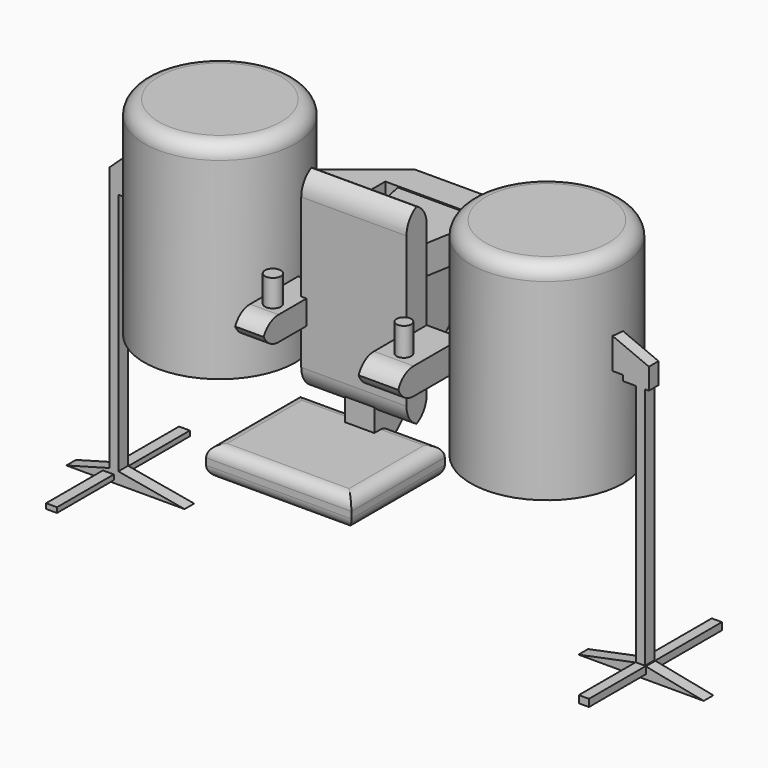
from build123d import *

# Parameters (mm, degrees)
F0_R         = 160.6336286285
F1_DEPTH     = 218.44
F0_R_2       = 159.7328245583
F3_DEPTH     = 63.5
F4_W         = 221.9782620668
F4_H         = 414.4903868437
F5_DEPTH     = 53.34
F6_T1_DEPTH  = 467.2623600039
F8_DEPTH     = 60.96
F4_W_2       = 306.4478710294
F4_H_2       = 62.861084938
F9_DEPTH     = 246.38
F10_R        = 24.5284097937
F11_W        = 61.5484267473
F11_H        = 264.6007202566
F12_DEPTH    = 287.782
F13_SIZE     = 205.74
F14_SIZE     = 81.28
F19_W        = 18.9964473248
F19_H        = 513.7299746275
F20_DEPTH    = 25.4
F21_W        = 22.9676365852
F21_H        = 10.7182264328
F22_DEPTH    = 175.26
F21_W_2      = 21.4364528656
F21_H_2      = 15.3118371964
F23_W        = 83.6651213467
F23_H        = 56.2124997377
F23_W_2      = 60.1342916489
F23_H_2      = 50.9834252298
F24_DEPTH    = 170.18
F25_T1_DEPTH = 274.7578773438
F25_T3_DEPTH = 298.2887070417
F26_R        = 30.6605122421
F26_2_R      = 30.6605122421
F27_R        = 16.7759014108
F28_DEPTH    = 93.722416088
F27_R_2      = 15.45819276


# Not quite as in the source:
# - a fillet or chamfer that OpenCascade refuses, or shapes differently, is made with other operations: its cross-section is extruded or revolved along the edge and cut away or added
# - the program builds the solid bodies; features that only make, move or delete a surface that nothing else refers to are left out


with BuildPart() as f1:
    # F0 (on Top) → F1 (new body, symmetric)
    with BuildSketch(Plane.XY):
        with Locations((167.6235944033, 0)):
            Circle(F0_R)
    extrude(amount=F1_DEPTH, both=True)

    # F26
    f26_edges = [f1.edges().sort_by_distance(p)[0] for p in [
        (6.989966, 0, 218.44),
    ]]
    fillet(f26_edges, radius=F26_R)


with BuildPart() as f1b:
    # F0 (on Top) → F1, piece 2 (new body, symmetric)
    with BuildSketch(Plane.XY):
        with Locations((-522.2776532173, 0)):
            Circle(F0_R_2)
    extrude(amount=F1_DEPTH, both=True)

    # F26#2
    f26_2_edges = [f1b.edges().sort_by_distance(p)[0] for p in [
        (-682.010478, 0, 218.44),
    ]]
    fillet(f26_2_edges, radius=F26_2_R)


with BuildPart() as f3:
    # F2 (on Top) → F3 (new body)
    with BuildSketch(Plane.XY):
        Polygon((-300.143301487, 237.2024357319), (-437.6519620419, 127.195507288), (-432.7409267426, 106.5692082047), (-312.0444483441, 106.5692082047), (-312.0444483441, 173.3591258526), (-42.8056791425, 173.3591258526), (-42.8056791425, 96.7471674085), (99.6140241623, 96.7471674085), (99.6140241623, 131.1243325472), (-56.5565414727, 237.2024357319), align=None)
    extrude(amount=F3_DEPTH)


with BuildPart() as f5:
    # F4 (on Front) → F5 (new body)
    with BuildSketch(Plane.XZ):
        with Locations((-197.0118135214, -29.95724231)):
            Rectangle(F4_W, F4_H)
    extrude(amount=F5_DEPTH)

    # F6: fillet of radius 49.0568195874 on 4 edges, made by hand

    # F6_s2 → F6_t1 (cut)
    with BuildSketch(Plane.YZ.offset(-430.6429935234)):
        with BuildLine():
            ThreePointArc((-49.0568195874, -237.2024357319), (-14.3684097937, -222.8340259382), (0, -188.1456161445))
            Line((0, -188.1456161445), (0, -237.2024357319))
            Line((0, -237.2024357319), (-49.0568195874, -237.2024357319))
        make_face()
        with BuildLine():
            ThreePointArc((-4.2831804126, -237.2024357319), (-38.9715902063, -222.8340259382), (-53.34, -188.1456161445))
            Line((-53.34, -188.1456161445), (-53.34, -237.2024357319))
            Line((-53.34, -237.2024357319), (-4.2831804126, -237.2024357319))
        make_face()
        with BuildLine():
            ThreePointArc((-4.2831804126, 177.2879511118), (-38.9715902063, 162.9195413181), (-53.34, 128.2311315244))
            Line((-53.34, 128.2311315244), (-53.34, 177.2879511118))
            Line((-53.34, 177.2879511118), (-4.2831804126, 177.2879511118))
        make_face()
        with BuildLine():
            ThreePointArc((-49.0568195874, 177.2879511118), (-14.3684097937, 162.9195413181), (0, 128.2311315244))
            Line((0, 128.2311315244), (0, 177.2879511118))
            Line((0, 177.2879511118), (-49.0568195874, 177.2879511118))
        make_face()
    extrude(amount=F6_T1_DEPTH, mode=Mode.SUBTRACT)

    # F23 (on Front) → F24 (join)
    with BuildSketch(Plane.XZ):
        with Locations((-53.6179151386, -87.4198973179)):
            Rectangle(F23_W, F23_H)
        with Locations((-326.8368244171, -82.1908283979)):
            Rectangle(F23_W_2, F23_H_2)
    extrude(amount=F24_DEPTH)

    # F25: fillet of radius 42.924717139 on 4 edges, made by hand

    # F25_s2 → F25_t1 (cut)
    with BuildSketch(Plane.YZ.offset(-464.215763089)):
        with BuildLine():
            ThreePointArc((-127.255282861, -56.699115783), (-157.6076414305, -69.2714743525), (-170.18, -99.623832922))
            Line((-170.18, -99.623832922), (-170.18, -56.699115783))
            Line((-170.18, -56.699115783), (-127.255282861, -56.699115783))
        make_face()
        with BuildLine():
            ThreePointArc((-127.255282861, -107.6825410128), (-157.6076414305, -95.1101824433), (-170.18, -64.7578238738))
            Line((-170.18, -64.7578238738), (-170.18, -107.6825410128))
            Line((-170.18, -107.6825410128), (-127.255282861, -107.6825410128))
        make_face()
    extrude(amount=F25_T1_DEPTH, mode=Mode.SUBTRACT)

    # F25_s4 → F25_t3 (cut)
    with BuildSketch(Plane.YZ.offset(-202.7622686594)):
        with BuildLine():
            ThreePointArc((-170.18, -102.238364588), (-157.6076414305, -71.8860060185), (-127.255282861, -59.313647449))
            Line((-127.255282861, -59.313647449), (-170.18, -59.313647449))
            Line((-170.18, -59.313647449), (-170.18, -102.238364588))
        make_face()
        with BuildLine():
            ThreePointArc((-127.255282861, -115.5261471868), (-157.6076414305, -102.9537886173), (-170.18, -72.6014300478))
            Line((-170.18, -72.6014300478), (-170.18, -115.5261471868))
            Line((-170.18, -115.5261471868), (-127.255282861, -115.5261471868))
        make_face()
    extrude(amount=F25_T3_DEPTH, mode=Mode.SUBTRACT)


with BuildPart() as f8:
    # F7 (on Top) → F8 (new body)
    with BuildSketch(Plane.XY):
        Polygon((-98.7913385034, 196.9104707241), (-290.3212606907, 192.9816454649), (-244.1576421261, -9.3525238335), (-134.1507136822, -9.3525238335), align=None)
    extrude(amount=F8_DEPTH)


with BuildPart() as f9:
    # F4 (on Front) → F9 (new body)
    with BuildSketch(Plane.XZ):
        with Locations((-201.0610103607, -299.5766699314)):
            Rectangle(F4_W_2, F4_H_2)
    extrude(amount=F9_DEPTH)

    # F10
    f10_edges = [f9.edges().sort_by_distance(p)[0] for p in [
        (-354.284946, -123.19, -268.146127),
        (-354.284946, -123.19, -331.007212),
        (-47.837075, -123.19, -268.146127),
        (-47.837075, -123.19, -331.007212),
        (-201.06101, -246.38, -268.146127),
        (-201.06101, -246.38, -331.007212),
        (-201.06101, 0, -268.146127),
        (-201.06101, 0, -331.007212),
    ]]
    fillet(f10_edges, radius=F10_R)


with BuildPart() as f12:
    # F11 (on Top) → F12 (new body)
    with BuildSketch(Plane.XY):
        with Locations((-194.3048760295, 91.1482293159)):
            Rectangle(F11_W, F11_H)
    extrude(amount=-F12_DEPTH)

    # F13
    f13_edges = [f12.edges().sort_by_distance(p)[0] for p in [
        (-194.304876, 223.448589, -287.782),
    ]]
    chamfer(f13_edges, length=F13_SIZE)

    # F14
    f14_edges = [f12.edges().sort_by_distance(p)[0] for p in [
        (-194.304876, 223.448589, -82.042),
    ]]
    chamfer(f14_edges, length=F14_SIZE)


with BuildPart() as f20:
    # F19 (on Front) → F20 (new body)
    with BuildSketch(Plane.XZ):
        Polygon((-662.3982787132, 0), (-672.3094582558, 90.7716751099), (-735.0803017616, 32.9563878477), (-735.0803017616, -11.643961072), (-716.0838544369, -11.643961072), (-697.0874071121, -11.643961072), (-697.0874071121, 0), align=None)
        with Locations((-725.5820780993, -268.5089483857)):
            Rectangle(F19_W, F19_H)
        Polygon((-716.0838544369, -525.3739356995), (-735.0803017616, -525.3739356995), (-825.9328603745, -550.1518845558), (-576.5013098717, -550.1518845558), align=None)
    extrude(amount=F20_DEPTH)


with BuildPart() as f20b:
    # F19 (on Front) → F20, piece 2 (new body)
    with BuildSketch(Plane.XZ):
        Polygon((403.0545651913, 32.9563878477), (320.4613029957, 67.6455572248), (305.5945038795, 0), (348.5430181026, 0), (348.5430181026, -11.643961072), (375.798791647, -11.643961072), (394.7952389717, -11.643961072), (403.0545651913, -11.643961072), align=None)
        with Locations((385.2970153093, -268.5089483857)):
            Rectangle(F19_W, F19_H)
        Polygon((518.6851024628, -550.1518845558), (394.7952389717, -525.3739356995), (375.798791647, -525.3739356995), (254.3867230415, -550.1518845558), align=None)
    extrude(amount=F20_DEPTH)


with BuildPart() as f22:
    # F21 (on Front) → F22 (new body, symmetric)
    with BuildSketch(Plane.XZ):
        with Locations((-737.2682392597, -539.6229028702)):
            Rectangle(F21_W, F21_H)
    extrude(amount=F22_DEPTH, both=True)


with BuildPart() as f22b:
    # F21 (on Front) → F22, piece 2 (new body, symmetric)
    with BuildSketch(Plane.XZ):
        with Locations((385.8506381512, -532.7326059341)):
            Rectangle(F21_W_2, F21_H_2)
    extrude(amount=F22_DEPTH, both=True)


with BuildPart() as f28:
    # F27 (on Top) → F28 (new body)
    with BuildSketch(Plane.XY):
        with Locations((-328.311920166, -102.629929781)):
            Circle(F27_R)
    extrude(amount=-F28_DEPTH)


with BuildPart() as f28b:
    # F27 (on Top) → F28, piece 2 (new body)
    with BuildSketch(Plane.XY):
        with Locations((-52.1512031555, -102.4584174156)):
            Circle(F27_R_2)
    extrude(amount=-F28_DEPTH)


solid = Compound([f1.part, f1b.part, f3.part, f5.part, f8.part, f9.part, f12.part, f20.part, f20b.part, f22.part, f22b.part, f28.part, f28b.part])
